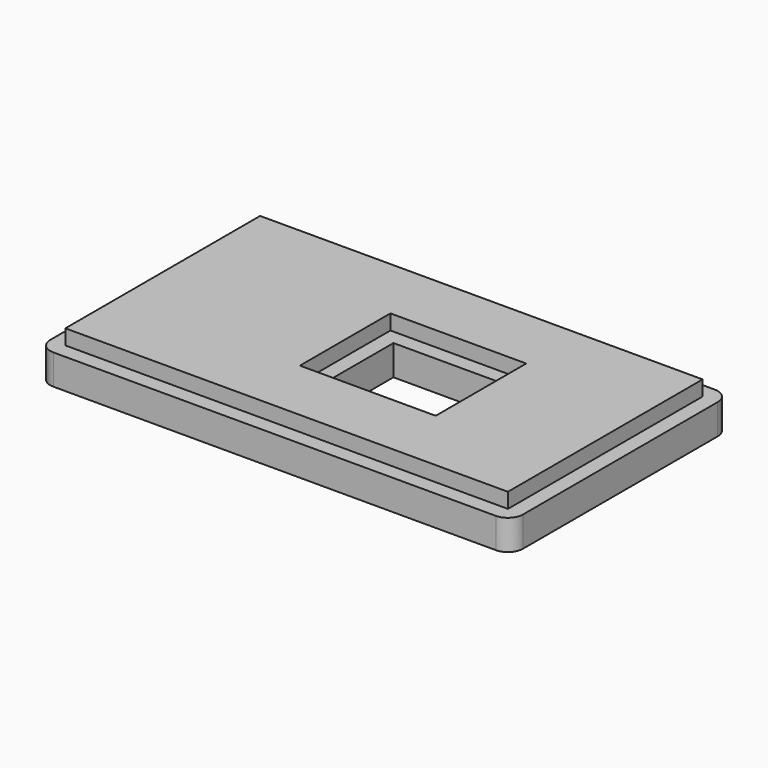
from build123d import *

# Parameters (mm, degrees)
F0_W        = 58.6601923168
F0_H        = 32.2631057742
F0_W_2      = 18
F0_H_2      = 15
F1_DEPTH    = 2
F2_T        = 2
F3_T1_DEPTH = 2
F3_T3_DEPTH = 14
F4_DEPTH    = 4


# Not quite as in the source:
# - a fillet or chamfer that OpenCascade refuses, or shapes differently, is made with other operations: its cross-section is extruded or revolved along the edge and cut away or added
# - a feature names something its author has since deleted; it is built from what else it names


with BuildPart() as f1:
    # F0 (on Top) → F1 (new body)
    with BuildSketch(Plane.XY):
        with Locations((-3.8516821679, 0)):
            Rectangle(F0_W, F0_H)
        Rectangle(F0_W_2, F0_H_2, mode=Mode.SUBTRACT)
    extrude(amount=F1_DEPTH)

    # F2
    f2_openings = [f1.faces().sort_by_distance(p)[0] for p in [
        (24.808942, 0, 2),
    ]]
    offset(amount=F2_T, openings=f2_openings, kind=Kind.INTERSECTION)

    # F3: fillet of radius 2 on 8 edges, made by hand

    # F3_s2 → F3_t1 (join)
    with BuildSketch(Plane.XY):
        with BuildLine():
            ThreePointArc((-31.1817783263, 16.1315528871), (-32.5959918887, 15.5457664495), (-33.1817783263, 14.1315528871))
            Line((-33.1817783263, 14.1315528871), (-33.1817783263, 16.1315528871))
            Line((-33.1817783263, 16.1315528871), (-31.1817783263, 16.1315528871))
        make_face()
        with BuildLine():
            ThreePointArc((-33.1817783263, -14.1315528871), (-32.5959918887, -15.5457664495), (-31.1817783263, -16.1315528871))
            Line((-31.1817783263, -16.1315528871), (-33.1817783263, -16.1315528871))
            Line((-33.1817783263, -16.1315528871), (-33.1817783263, -14.1315528871))
        make_face()
        with BuildLine():
            ThreePointArc((25.4784139905, -14.1315528871), (24.8926275528, -15.5457664495), (23.4784139905, -16.1315528871))
            Line((23.4784139905, -16.1315528871), (25.4784139905, -16.1315528871))
            Line((25.4784139905, -16.1315528871), (25.4784139905, -14.1315528871))
        make_face()
        with BuildLine():
            ThreePointArc((25.4784139905, 14.1315528871), (24.8926275528, 15.5457664495), (23.4784139905, 16.1315528871))
            Line((23.4784139905, 16.1315528871), (25.4784139905, 16.1315528871))
            Line((25.4784139905, 16.1315528871), (25.4784139905, 14.1315528871))
        make_face()
    extrude(amount=F3_T1_DEPTH)

    # F3_s4 → F3_t3 (cut)
    with BuildSketch(Plane.XY.offset(-7)):
        with BuildLine():
            ThreePointArc((25.4784139905, -18.1315528871), (26.8926275528, -17.5457664495), (27.4784139905, -16.1315528871))
            Line((27.4784139905, -16.1315528871), (27.4784139905, -18.1315528871))
            Line((27.4784139905, -18.1315528871), (25.4784139905, -18.1315528871))
        make_face()
        with BuildLine():
            ThreePointArc((27.4784139905, 16.1315528871), (26.8926275528, 17.5457664495), (25.4784139905, 18.1315528871))
            Line((25.4784139905, 18.1315528871), (27.4784139905, 18.1315528871))
            Line((27.4784139905, 18.1315528871), (27.4784139905, 16.1315528871))
        make_face()
        with BuildLine():
            ThreePointArc((-35.1817783263, 16.1315528871), (-34.5959918887, 17.5457664495), (-33.1817783263, 18.1315528871))
            Line((-33.1817783263, 18.1315528871), (-35.1817783263, 18.1315528871))
            Line((-35.1817783263, 18.1315528871), (-35.1817783263, 16.1315528871))
        make_face()
        with BuildLine():
            ThreePointArc((-35.1817783263, -16.1315528871), (-34.5959918887, -17.5457664495), (-33.1817783263, -18.1315528871))
            Line((-33.1817783263, -18.1315528871), (-35.1817783263, -18.1315528871))
            Line((-35.1817783263, -18.1315528871), (-35.1817783263, -16.1315528871))
        make_face()
    extrude(amount=F3_T3_DEPTH, mode=Mode.SUBTRACT)

    # F0 (on Top) → F4 (join)
    with BuildSketch(Plane.XY):
        with Locations((-3.8516821679, 0)):
            Rectangle(F0_W, F0_H)
        Rectangle(F0_W_2, F0_H_2, mode=Mode.SUBTRACT)
    extrude(amount=F4_DEPTH)


solid = f1.part
